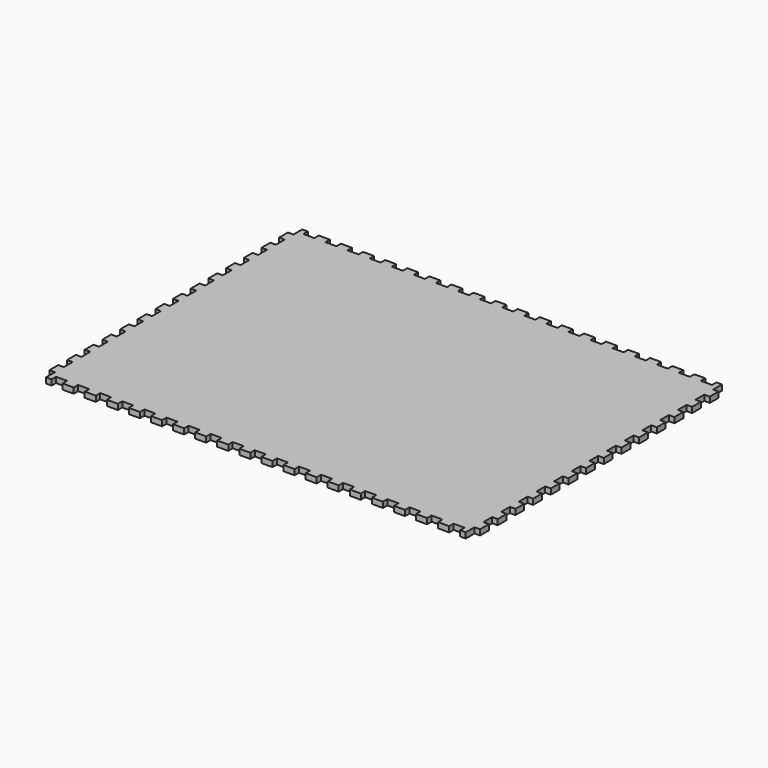
from build123d import *

# Parameters (mm, degrees)
F1_DEPTH = 2.5


# Not quite as in the source:
# - ends of sketch curves that miss each other by under 0.0002 mm in the source are joined


with BuildPart() as f1:
    # F0 (on Top) → F1 (new body, symmetric)
    with BuildSketch(Plane.XY):
        Polygon((-189.0456426144, -116.6238892078), (-189.0456426144, -126.6238892078), (-184.0456426144, -126.6238850355), (-184.0456426144, -136.6238850355), (-179.0456426144, -136.6238850355), (-179.0456426144, -131.6238850355), (-169.0456426144, -131.6238850355), (-169.0456426144, -136.6238850355), (-159.0456426144, -136.6238850355), (-159.0456426144, -131.6238850355), (-149.0456426144, -131.6238850355), (-149.0456426144, -136.6238850355), (-139.0456426144, -136.6238850355), (-139.0456426144, -131.6238850355), (-129.0456426144, -131.6238850355), (-129.0456426144, -136.6238850355), (-119.0456426144, -136.6238850355), (-119.0456426144, -131.6238850355), (-109.0456426144, -131.6238850355), (-109.0456426144, -136.6238850355), (-99.0456426144, -136.6238850355), (-99.0456426144, -131.6238850355), (-89.0456426144, -131.6238850355), (-89.0456426144, -136.6238850355), (-79.0456426144, -136.6238850355), (-79.0456426144, -131.6238850355), (-69.0456426144, -131.6238850355), (-69.0456426144, -136.6238850355), (-59.0456426144, -136.6238850355), (-59.0456426144, -131.6238850355), (-49.0456426144, -131.6238850355), (-49.0456426144, -136.6238850355), (-39.0456426144, -136.6238850355), (-39.0456426144, -131.6238850355), (-29.0456426144, -131.6238850355), (-29.0456426144, -136.6238850355), (-19.0456426144, -136.6238850355), (-19.0456426144, -131.6238850355), (-9.0456426144, -131.6238850355), (-9.0456426144, -136.6238850355), (0.9543573856, -136.6238850355), (0.9543573856, -131.6238850355), (10.9543573856, -131.6238850355), (10.9543573856, -136.6238850355), (20.9543573856, -136.6238850355), (20.9543573856, -131.6238850355), (30.9543573856, -131.6238850355), (30.9543573856, -136.6238850355), (40.9543573856, -136.6238850355), (40.9543573856, -131.6238850355), (50.9543573856, -131.6238850355), (50.9543573856, -136.6238850355), (60.9543573856, -136.6238850355), (60.9543573856, -131.6238850355), (70.9543573856, -131.6238850355), (70.9543573856, -136.6238850355), (80.9543573856, -136.6238850355), (80.9543573856, -131.6238850355), (90.9543573856, -131.6238850355), (90.9543573856, -136.6238850355), (100.9543573856, -136.6238850355), (100.9543573856, -131.6238850355), (110.9543573856, -131.6238850355), (110.9543573856, -136.6238850355), (120.9543573856, -136.6238850355), (120.9543573856, -131.6238850355), (130.9543573856, -131.6238850355), (130.9543573856, -136.6238850355), (140.9543573856, -136.6238850355), (140.9543573856, -131.6238850355), (150.9543573856, -131.6238850355), (150.9543573856, -136.6238850355), (160.9543573856, -136.6238850355), (160.9543573856, -131.6238850355), (170.9543573856, -131.6238850355), (170.9543573856, -136.6238850355), (180.9543573856, -136.6238850355), (180.9543573856, -131.6238850355), (190.9543573856, -131.6238850355), (190.9543573856, -136.6238850355), (195.9543573856, -136.6238850355), (195.9543573856, -126.6238850355), (200.9543573856, -126.6238850355), (200.9543502331, -116.6238892078), (195.9543502331, -116.6238892078), (195.9543502331, -106.6238892078), (200.9543502331, -106.6238892078), (200.9543502331, -96.6238892078), (195.9543502331, -96.6238892078), (195.9543502331, -86.6238892078), (200.9543502331, -86.6238892078), (200.9543502331, -76.6238892078), (195.9543502331, -76.6238892078), (195.9543502331, -66.6238892078), (200.9543502331, -66.6238892078), (200.9543502331, -56.6238892078), (195.9543502331, -56.6238892078), (195.9543502331, -46.6238892078), (200.9543573856, -46.6238892078), (200.9543573856, -36.6238892078), (195.9543573856, -36.6238892078), (195.9543573856, -26.6238892078), (200.9543502331, -26.6238892078), (200.9543502331, -16.6238892078), (195.9543502331, -16.6238892078), (195.9543502331, -6.6238892078), (200.9543502331, -6.6238892078), (200.9543502331, 3.3761107922), (195.9543502331, 3.3761107922), (195.9543502331, 13.3761107922), (200.9543502331, 13.3761107922), (200.9543502331, 23.3761107922), (195.9543502331, 23.3761107922), (195.9543502331, 33.3761107922), (200.9543502331, 33.3761107922), (200.9543502331, 43.3761107922), (195.9543502331, 43.3761107922), (195.9543502331, 53.3761107922), (200.9543502331, 53.3761107922), (200.9543502331, 63.3761107922), (195.9543502331, 63.3761107922), (195.9543502331, 73.3761107922), (200.9543502331, 73.3761107922), (200.9543502331, 83.3761107922), (195.9543502331, 83.3761107922), (195.9543502331, 93.3761107922), (200.9543502331, 93.3761107922), (200.9543502331, 103.3761107922), (195.9543502331, 103.3761107922), (195.9543502331, 113.3761107922), (200.9543502331, 113.3761107922), (200.9543502331, 123.3761107922), (195.9543502331, 123.3761107922), (195.9543502331, 133.3761107922), (200.9543502331, 133.3761107922), (200.9543502331, 143.3761107922), (195.9543573856, 143.3761107922), (195.9543573856, 153.3761107922), (190.9543573856, 153.3761107922), (190.9543573856, 148.3761107922), (180.9543573856, 148.3761107922), (180.9543573856, 153.3761107922), (170.9543573856, 153.3761107922), (170.9543573856, 148.3761107922), (160.9543573856, 148.3761107922), (160.9543573856, 153.3761107922), (150.9543573856, 153.3761107922), (150.9543573856, 148.3761107922), (140.9543573856, 148.3761107922), (140.9543573856, 153.3761107922), (130.9543573856, 153.3761107922), (130.9543573856, 148.3761107922), (120.9543573856, 148.3761107922), (120.9543573856, 153.3761107922), (110.9543573856, 153.3761107922), (110.9543573856, 148.3761107922), (100.9543573856, 148.3761107922), (100.9543573856, 153.3761107922), (90.9543573856, 153.3761107922), (90.9543573856, 148.3761107922), (80.9543573856, 148.3761107922), (80.9543573856, 153.3761107922), (70.9543573856, 153.3761107922), (70.9543573856, 148.3761107922), (60.9543573856, 148.3761107922), (60.9543573856, 153.3761107922), (50.9543573856, 153.3761107922), (50.9543573856, 148.3761107922), (40.9543573856, 148.3761107922), (40.9543573856, 153.3761107922), (30.9543573856, 153.3761107922), (30.9543573856, 148.3761107922), (20.9543573856, 148.3761107922), (20.9543573856, 153.3761107922), (10.9543573856, 153.3761107922), (10.9543573856, 148.3761107922), (0.9543573856, 148.3761107922), (0.9543573856, 153.3761107922), (-9.0456426144, 153.3761107922), (-9.0456426144, 148.3761107922), (-19.0456426144, 148.3761107922), (-19.0456426144, 153.3761107922), (-29.0456426144, 153.3761107922), (-29.0456426144, 148.3761107922), (-39.0456426144, 148.3761107922), (-39.0456426144, 153.3761107922), (-49.0456426144, 153.3761107922), (-49.0456426144, 148.3761107922), (-59.0456426144, 148.3761107922), (-59.0456426144, 153.3761107922), (-69.0456426144, 153.3761107922), (-69.0456426144, 148.3761107922), (-79.0456426144, 148.3761107922), (-79.0456426144, 153.3761107922), (-89.0456426144, 153.3761107922), (-89.0456426144, 148.3761107922), (-99.0456426144, 148.3761107922), (-99.0456426144, 153.3761107922), (-109.0456426144, 153.3761107922), (-109.0456426144, 148.3761107922), (-119.0456426144, 148.3761107922), (-119.0456426144, 153.3761107922), (-129.0456426144, 153.3761107922), (-129.0456426144, 148.3761107922), (-139.0456426144, 148.3761107922), (-139.0456426144, 153.3761107922), (-149.0456426144, 153.3761107922), (-149.0456426144, 148.3761107922), (-159.0456426144, 148.3761107922), (-159.0456426144, 153.3761107922), (-169.0456426144, 153.3761107922), (-169.0456426144, 148.3761107922), (-179.0456426144, 148.3761107922), (-179.0456426144, 153.3761107922), (-184.0456426144, 153.3761107922), (-184.0456426144, 143.3761107922), (-189.0456426144, 143.3761107922), (-189.0456426144, 133.3761107922), (-184.0456426144, 133.3761107922), (-184.0456426144, 123.3761107922), (-189.0456426144, 123.3761107922), (-189.0456426144, 113.3761107922), (-184.0456426144, 113.3761107922), (-184.0456426144, 103.3761107922), (-189.0456426144, 103.3761107922), (-189.0456426144, 93.3761107922), (-184.0456426144, 93.3761107922), (-184.0456426144, 83.3761107922), (-189.0456426144, 83.3761107922), (-189.0456426144, 73.3761107922), (-184.0456426144, 73.3761107922), (-184.0456426144, 63.3761107922), (-189.0456426144, 63.3761107922), (-189.0456426144, 53.3761107922), (-184.0456426144, 53.3761107922), (-184.0456426144, 43.3761107922), (-189.0456426144, 43.3761107922), (-189.0456426144, 33.3761107922), (-184.0456426144, 33.3761107922), (-184.0456426144, 23.3761107922), (-189.0456426144, 23.3761107922), (-189.0456426144, 13.3761107922), (-184.0456426144, 13.3761107922), (-184.0456426144, 3.3761107922), (-189.0456426144, 3.3761107922), (-189.0456426144, -6.6238892078), (-184.0456426144, -6.6238892078), (-184.0456426144, -16.6238892078), (-189.0456426144, -16.6238892078), (-189.0456426144, -26.6238892078), (-184.0456426144, -26.6238892078), (-184.0456426144, -36.6238892078), (-189.0456426144, -36.6238892078), (-189.0456426144, -46.6238892078), (-184.0456426144, -46.6238892078), (-184.0456426144, -56.6238892078), (-189.0456426144, -56.6238892078), (-189.0456426144, -66.6238892078), (-184.0456426144, -66.6238892078), (-184.0456426144, -76.6238892078), (-189.0456426144, -76.6238892078), (-189.0456426144, -86.6238892078), (-184.0456426144, -86.6238892078), (-184.0456426144, -96.6238892078), (-189.0456426144, -96.6238892078), (-189.0456426144, -106.6238892078), (-184.0456426144, -106.6238892078), (-184.0456426144, -116.6238892078), align=None)
    extrude(amount=F1_DEPTH, both=True)


solid = f1.part
